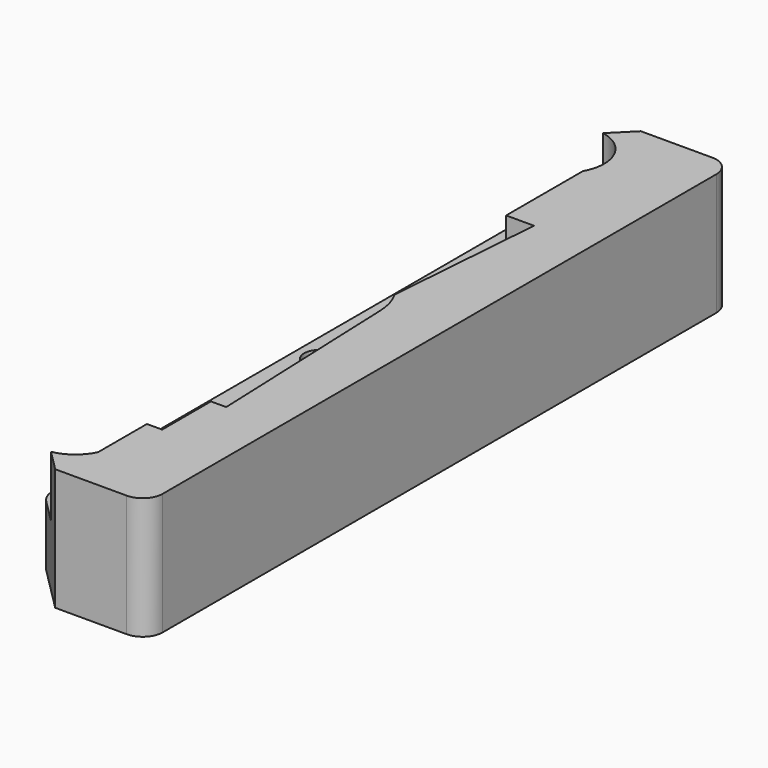
from build123d import *

# Parameters (mm, degrees)
F0_R     = 6.35
F1_DEPTH = 50.8
F2_R     = 8.334375
F4_DEPTH = 25.4
F6_DEPTH = 25.4


with BuildPart() as f1:
    # F0 (on Top) → F1 (new body)
    with BuildSketch(Plane.XY):
        with BuildLine():
            Line((-21.4546158184, 127), (-21.4546158184, -127))
            ThreePointArc((-21.4546158184, -127), (-20.7295683656, -130.6450596933), (-18.6648079092, -133.7351920908))
            Line((-18.6648079092, -133.7351920908), (0, -152.4))
            Line((0, -152.4), (38.1, -152.4))
            Line((38.1, -152.4), (38.1, 152.4))
            Line((38.1, 152.4), (0, 152.4))
            Line((0, 152.4), (-18.6648079092, 133.7351920908))
            ThreePointArc((-18.6648079092, 133.7351920908), (-20.7295683656, 130.6450596933), (-21.4546158184, 127))
        make_face()
        with Locations((-11.9296158184, -127)):
            Circle(F0_R, mode=Mode.SUBTRACT)
        with Locations((-11.9296158184, 0)):
            Circle(F0_R, mode=Mode.SUBTRACT)
        with Locations((-11.9296158184, 127)):
            Circle(F0_R, mode=Mode.SUBTRACT)
    extrude(amount=F1_DEPTH)

    # F2
    f2_edges = [f1.edges().sort_by_distance(p)[0] for p in [
        (38.1, 152.4, 25.4),
        (38.1, -152.4, 25.4),
    ]]
    fillet(f2_edges, radius=F2_R)

    # F3 (on face) → F4 (cut)
    with BuildSketch(Plane.XY.offset(50.8)):
        with BuildLine():
            Line((-18.6648079092, -133.7351920908), (-8.741865195, -143.658134805))
            ThreePointArc((-8.741865195, -143.658134805), (-1.565286118, -140.4251956813), (3.379023496, -134.3007377408))
            Line((3.379023496, -134.3007377408), (3.379023496, -83.5007377408))
            Line((3.379023496, -83.5007377408), (16.079023496, -83.5007377408))
            Line((16.079023496, -83.5007377408), (12.7517639776, 0.9721621486))
            ThreePointArc((12.7517639776, 0.9721621486), (11.7712856877, 6.9557800194), (9.3626122843, 12.5202488115))
            Line((9.3626122843, 12.5202488115), (14.4614139572, 78.7273198366))
            Line((14.4614139572, 78.7273198366), (2.8423227302, 78.7273198366))
            Line((2.8423227302, 78.7273198366), (2.8423227302, 118.6666308892))
            ThreePointArc((2.8423227302, 118.6666308892), (3.4580879019, 134.1325860273), (-8.741865195, 143.658134805))
            Line((-8.741865195, 143.658134805), (-18.6648079092, 133.7351920908))
            ThreePointArc((-18.6648079092, 133.7351920908), (-20.7295683656, 130.6450596933), (-21.4546158184, 127))
            Line((-21.4546158184, 127), (-21.4546158184, -127))
            ThreePointArc((-21.4546158184, -127), (-20.7295683656, -130.6450596933), (-18.6648079092, -133.7351920908))
        make_face()
    extrude(amount=-F4_DEPTH, mode=Mode.SUBTRACT)

    # F5 (on face) → F6 (cut)
    with BuildSketch(Plane(origin=(0, -83.5007377408, 0), x_dir=(-1, 0, 0), z_dir=(0, 1, 0))):
        Polygon((-3.379023496, 50.8), (-9.729023496, 50.8), (-9.729023496, 45.24375), (-8.935273496, 45.24375), (-8.935273496, 44.45), (-8.141523496, 44.45), (-8.141523496, 43.65625), (-4.966523496, 43.65625), (-4.966523496, 44.45), (-4.172773496, 44.45), (-4.172773496, 45.24375), (-3.379023496, 45.24375), align=None)
    extrude(amount=-F6_DEPTH, mode=Mode.SUBTRACT)


solid = f1.part
